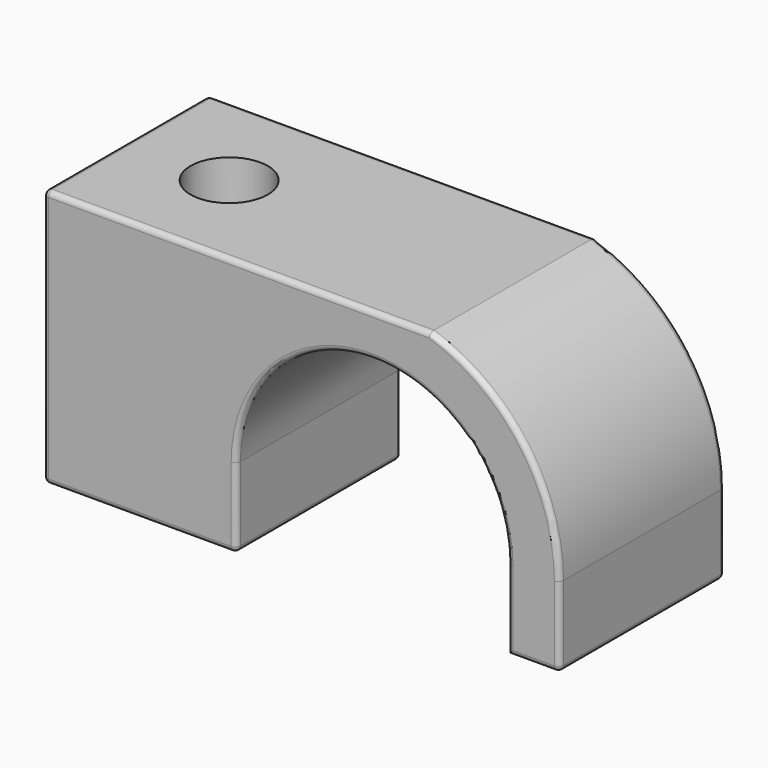
from build123d import *

# Parameters (mm, degrees)
F1_DEPTH = 4
F3_R     = 0.1
F2_R     = 0.75
F4_DEPTH = 25


# Not quite as in the source:
# - ends of sketch curves that miss each other by under 0.0002 mm in the source are joined


with BuildPart() as f1:
    # F0 (on Front) → F1 (new body)
    with BuildSketch(Plane.XZ):
        with BuildLine():
            Line((0, 5), (0, 0))
            Line((0, 0), (3.7373243831, 0))
            Line((3.7373243831, 0), (3.7373243831, 1.5373318456))
            ThreePointArc((3.7373243831, 1.5373318456), (6.3598005329, 4.1775164411), (8.9999850781, 1.5550552132))
            Line((8.9999850781, 1.5550552132), (9, 1.5461935545))
            Line((9, 1.5461935545), (9, 0))
            Line((9, 0), (9.6543736474, 0))
            ThreePointArc((9.6543736474, 0), (9.9125401886, 0.7540174245), (10, 1.5461935545))
            ThreePointArc((10, 1.5461935545), (9.3062869056, 3.680900869), (7.4901947663, 5))
            Line((7.4901947663, 5), (5.2471296168, 5))
            Line((5.2471296168, 5), (0, 5))
        make_face()
        with BuildLine():
            Line((10, 0), (10, 1.5461935545))
            ThreePointArc((10, 1.5461935545), (9.9125401886, 0.7540174245), (9.6543736474, 0))
            Line((9.6543736474, 0), (10, 0))
        make_face()
    extrude(amount=F1_DEPTH)

    # F3
    f3_edges = [f1.edges().sort_by_distance(p)[0] for p in [
        (3.745097, -4, 5),
        (0, -2, 5),
        (0, -4, 2.5),
        (6.359793, -4, 4.177516),
        (3.737324, -2, 0),
        (1.868662, -4, 0),
        (9.5, -4, 0),
        (10, -2, 0),
        (9.5, 0, 0),
        (10, 0, 0.773097),
        (10, -4, 0.773097),
        (3.737324, 0, 0.768666),
        (3.745097, 0, 5),
        (0, 0, 2.5),
        (1.868662, 0, 0),
        (0, -2, 0),
    ]]
    fillet(f3_edges, radius=F3_R)

    # F2 (on face) → F4 (cut)
    with BuildSketch(Plane.XY.offset(5)):
        with Locations((2, -2)):
            Circle(F2_R)
    extrude(amount=-F4_DEPTH, mode=Mode.SUBTRACT)


solid = f1.part
